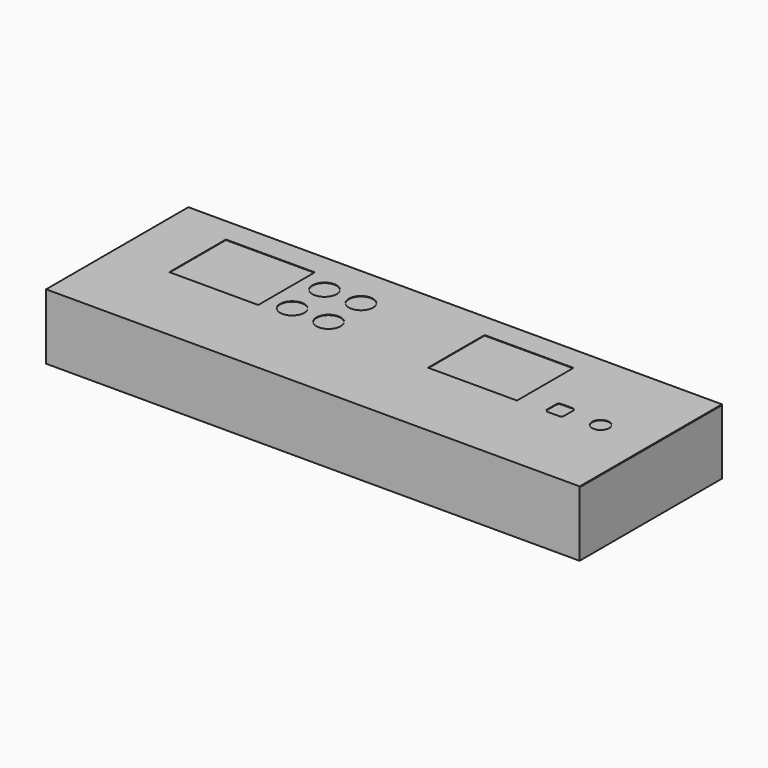
from build123d import *

# Parameters (mm, degrees)
F1_DEPTH = 209.55
F2_W     = 69.85
F2_H     = 55.5625
F3_DEPTH = 0.4064


# Not quite as in the source:
# - the dataset's text gives a spline's control points without its knots; the knots are read off the source's solid


with BuildPart() as f1:
    # F0 (on Right) → F1 (new body, symmetric)
    with BuildSketch(Plane.YZ):
        Polygon((-139.7, 0), (0, 0), (0, 50.8), (-139.2936, 50.8), (-139.2936, 51.054), (0, 51.054), (0, 51.4604), (-139.7, 51.4604), align=None)
    extrude(amount=F1_DEPTH, both=True)

    # F2 (on face) → F3 (cut, through all)
    with BuildSketch(Plane.XY.offset(51.4604)):
        with Locations((-129.8449253923, -46.8822261976)):
            Rectangle(F2_W, F2_H)
        Polygon((108.2948828077, -19.1009761976), (38.4448828077, -19.1009761976), (38.4448828077, -74.6634761976), (108.2948828077, -74.6634761976), (108.2948828077, -68.4133743976), (108.2948828077, -42.0156877976), align=None)
        with BuildLine():
            add(Edge.make_bspline(
                [(130.8209744077, -61.8670069976), (130.3807162077, -62.3079763976), (130.1230078077, -62.9274315976), (130.1230078077, -63.5509761976)],
                knots=[1, 1, 1, 1, 2, 2, 2, 2], degree=3))
            Line((130.1230078077, -63.5509761976), (130.1230078077, -72.2822261976))
            add(Edge.make_bspline(
                [(130.1230078077, -72.2822261976), (130.1230078077, -72.9057961976), (130.3807162077, -73.5252259976), (130.8209744077, -73.9654841976)],
                knots=[0, 0, 0, 0, 1, 1, 1, 1], degree=3))
            add(Edge.make_bspline(
                [(130.8209744077, -73.9654841976), (131.2619438077, -74.4064789976), (131.8813990077, -74.6634761976), (132.5042578077, -74.6634761976)],
                knots=[1, 1, 1, 1, 2, 2, 2, 2], degree=3))
            Line((132.5042578077, -74.6634761976), (141.2355078077, -74.6634761976))
            add(Edge.make_bspline(
                [(141.2355078077, -74.6634761976), (141.8597382077, -74.6634761976), (142.4784822077, -74.4064789976), (142.9194516077, -73.9654841976)],
                knots=[0, 0, 0, 0, 1, 1, 1, 1], degree=3))
            add(Edge.make_bspline(
                [(142.9194516077, -73.9654841976), (143.3604210077, -73.5252259976), (143.6167578077, -72.9057961976), (143.6167578077, -72.2822261976)],
                knots=[1, 1, 1, 1, 2, 2, 2, 2], degree=3))
            Line((143.6167578077, -72.2822261976), (143.6167578077, -63.5509761976))
            add(Edge.make_bspline(
                [(143.6167578077, -63.5509761976), (143.6167578077, -62.9274315976), (143.3604210077, -62.3079763976), (142.9194516077, -61.8670069976), (142.4784822077, -61.4260375976), (141.8597382077, -61.1697261976), (141.2355078077, -61.1697261976)],
                knots=[0, 0, 0, 0, 1, 1, 1, 2, 2, 2, 2], degree=3))
            Line((141.2355078077, -61.1697261976), (132.5042578077, -61.1697261976))
            add(Edge.make_bspline(
                [(132.5042578077, -61.1697261976), (131.8813990077, -61.1697261976), (131.2619438077, -61.4260375976), (130.8209744077, -61.8670069976)],
                knots=[0, 0, 0, 0, 1, 1, 1, 1], degree=3))
        make_face()
        with BuildLine():
            add(Edge.make_bspline(
                [(-69.1344295923, -26.6533105976), (-70.8976467923, -24.8901187976), (-73.3763565923, -23.8634761976), (-75.8699253923, -23.8634761976)],
                knots=[7, 7, 7, 7, 8, 8, 8, 8], degree=3))
            add(Edge.make_bspline(
                [(-75.8699253923, -23.8634761976), (-78.3631639923, -23.8634761976), (-80.8419245923, -24.8901187976), (-82.6050909923, -26.6533105976), (-84.3682827923, -28.4165277976), (-85.3949253923, -30.8949327976), (-85.3949253923, -33.3884761976), (-85.3949253923, -35.8820449976), (-84.3682827923, -38.3604499976), (-82.6050909923, -40.1236163976)],
                knots=[0, 0, 0, 0, 1, 1, 1, 2, 2, 2, 3, 3, 3, 3], degree=3))
            add(Edge.make_bspline(
                [(-82.6050909923, -40.1236163976), (-80.8419245923, -41.8868589976), (-78.3631639923, -42.9134761976), (-75.8699253923, -42.9134761976), (-73.3763565923, -42.9134761976), (-70.8976467923, -41.8868589976), (-69.1344295923, -40.1236163976)],
                knots=[3, 3, 3, 3, 4, 4, 4, 5, 5, 5, 5], degree=3))
            add(Edge.make_bspline(
                [(-69.1344295923, -40.1236163976), (-67.3712377923, -38.3604499976), (-66.3449253923, -35.8820449976), (-66.3449253923, -33.3884761976), (-66.3449253923, -30.8949327976), (-67.3712377923, -28.4165277976), (-69.1344295923, -26.6533105976)],
                knots=[5, 5, 5, 5, 6, 6, 6, 7, 7, 7, 7], degree=3))
        make_face()
        with BuildLine():
            add(Edge.make_bspline(
                [(-69.1344295923, -58.4033105976), (-70.8976467923, -56.6401187976), (-73.3763565923, -55.6134761976), (-75.8699253923, -55.6134761976)],
                knots=[7, 7, 7, 7, 8, 8, 8, 8], degree=3))
            add(Edge.make_bspline(
                [(-75.8699253923, -55.6134761976), (-78.3631639923, -55.6134761976), (-80.8419245923, -56.6401187976), (-82.6050909923, -58.4033105976), (-84.3682827923, -60.1665277976), (-85.3949253923, -62.6449327976), (-85.3949253923, -65.1384761976), (-85.3949253923, -67.6320449976), (-84.3682827923, -70.1104499976), (-82.6050909923, -71.8736163976)],
                knots=[0, 0, 0, 0, 1, 1, 1, 2, 2, 2, 3, 3, 3, 3], degree=3))
            add(Edge.make_bspline(
                [(-82.6050909923, -71.8736163976), (-80.8419245923, -73.6368589976), (-78.3631639923, -74.6634761976), (-75.8699253923, -74.6634761976), (-73.3763565923, -74.6634761976), (-70.8976467923, -73.6368589976), (-69.1344295923, -71.8736163976)],
                knots=[3, 3, 3, 3, 4, 4, 4, 5, 5, 5, 5], degree=3))
            add(Edge.make_bspline(
                [(-69.1344295923, -71.8736163976), (-67.3712377923, -70.1104499976), (-66.3449253923, -67.6320449976), (-66.3449253923, -65.1384761976), (-66.3449253923, -62.6449327976), (-67.3712377923, -60.1665277976), (-69.1344295923, -58.4033105976)],
                knots=[5, 5, 5, 5, 6, 6, 6, 7, 7, 7, 7], degree=3))
        make_face()
        with BuildLine():
            add(Edge.make_bspline(
                [(-40.5442911923, -58.4033105976), (-42.3074575923, -56.6401187976), (-44.7858879923, -55.6134761976), (-47.2794567923, -55.6134761976)],
                knots=[7, 7, 7, 7, 8, 8, 8, 8], degree=3))
            add(Edge.make_bspline(
                [(-47.2794567923, -55.6134761976), (-49.7733303923, -55.6134761976), (-52.2517353923, -56.6401187976), (-54.0149271923, -58.4033105976), (-55.7781443923, -60.1665277976), (-56.8044567923, -62.6449327976), (-56.8044567923, -65.1384761976), (-56.8044567923, -67.6320449976), (-55.7781443923, -70.1104499976), (-54.0149271923, -71.8736163976)],
                knots=[0, 0, 0, 0, 1, 1, 1, 2, 2, 2, 3, 3, 3, 3], degree=3))
            add(Edge.make_bspline(
                [(-54.0149271923, -71.8736163976), (-52.2517353923, -73.6368589976), (-49.7733303923, -74.6634761976), (-47.2794567923, -74.6634761976), (-44.7858879923, -74.6634761976), (-42.3074575923, -73.6368589976), (-40.5442911923, -71.8736163976)],
                knots=[3, 3, 3, 3, 4, 4, 4, 5, 5, 5, 5], degree=3))
            add(Edge.make_bspline(
                [(-40.5442911923, -71.8736163976), (-38.7807183923, -70.1104499976), (-37.7547615923, -67.6320449976), (-37.7547615923, -65.1384761976), (-37.7547615923, -62.6449327976), (-38.7807183923, -60.1665277976), (-40.5442911923, -58.4033105976)],
                knots=[5, 5, 5, 5, 6, 6, 6, 7, 7, 7, 7], degree=3))
        make_face()
        with BuildLine():
            add(Edge.make_bspline(
                [(-40.5442911923, -26.6533105976), (-42.3074575923, -24.8901187976), (-44.7858879923, -23.8634761976), (-47.2794567923, -23.8634761976)],
                knots=[7, 7, 7, 7, 8, 8, 8, 8], degree=3))
            add(Edge.make_bspline(
                [(-47.2794567923, -23.8634761976), (-49.7733303923, -23.8634761976), (-52.2517353923, -24.8901187976), (-54.0149271923, -26.6533105976), (-55.7781443923, -28.4165277976), (-56.8044567923, -30.8949327976), (-56.8044567923, -33.3884761976), (-56.8044567923, -35.8820449976), (-55.7781443923, -38.3604499976), (-54.0149271923, -40.1236163976)],
                knots=[0, 0, 0, 0, 1, 1, 1, 2, 2, 2, 3, 3, 3, 3], degree=3))
            add(Edge.make_bspline(
                [(-54.0149271923, -40.1236163976), (-52.2517353923, -41.8868589976), (-49.7733303923, -42.9134761976), (-47.2794567923, -42.9134761976), (-44.7858879923, -42.9134761976), (-42.3074575923, -41.8868589976), (-40.5442911923, -40.1236163976)],
                knots=[3, 3, 3, 3, 4, 4, 4, 5, 5, 5, 5], degree=3))
            add(Edge.make_bspline(
                [(-40.5442911923, -40.1236163976), (-38.7807183923, -38.3604499976), (-37.7547615923, -35.8820449976), (-37.7547615923, -33.3884761976), (-37.7547615923, -30.8949327976), (-38.7807183923, -28.4165277976), (-40.5442911923, -26.6533105976)],
                knots=[5, 5, 5, 5, 6, 6, 6, 7, 7, 7, 7], degree=3))
        make_face()
        with BuildLine():
            add(Edge.make_bspline(
                [(173.3906378077, -63.1458461976), (172.1421516077, -61.8966487976), (170.3872148077, -61.1697261976), (168.6198828077, -61.1697261976)],
                knots=[7, 7, 7, 7, 8, 8, 8, 8], degree=3))
            add(Edge.make_bspline(
                [(168.6198828077, -61.1697261976), (166.8539224077, -61.1697261976), (165.0989856077, -61.8966487976), (163.8497882077, -63.1458461976)],
                knots=[0, 0, 0, 0, 1, 1, 1, 1], degree=3))
            add(Edge.make_bspline(
                [(163.8497882077, -63.1458461976), (162.6006162077, -64.3943577976), (161.8730078077, -66.1499549976), (161.8730078077, -67.9166011976), (161.8730078077, -69.6825615976), (162.6006162077, -71.4381841976), (163.8497882077, -72.6873815976)],
                knots=[1, 1, 1, 1, 2, 2, 2, 3, 3, 3, 3], degree=3))
            add(Edge.make_bspline(
                [(163.8497882077, -72.6873815976), (165.0989856077, -73.9358677976), (166.8539224077, -74.6634761976), (168.6198828077, -74.6634761976), (170.3872148077, -74.6634761976), (172.1421516077, -73.9358677976), (173.3906378077, -72.6873815976)],
                knots=[3, 3, 3, 3, 4, 4, 4, 5, 5, 5, 5], degree=3))
            add(Edge.make_bspline(
                [(173.3906378077, -72.6873815976), (174.6398098077, -71.4381841976), (175.3667578077, -69.6825615976), (175.3667578077, -67.9166011976), (175.3667578077, -66.1499549976), (174.6398098077, -64.3943577976), (173.3906378077, -63.1458461976)],
                knots=[5, 5, 5, 5, 6, 6, 6, 7, 7, 7, 7], degree=3))
        make_face()
    extrude(amount=-F3_DEPTH, mode=Mode.SUBTRACT)


solid = f1.part
